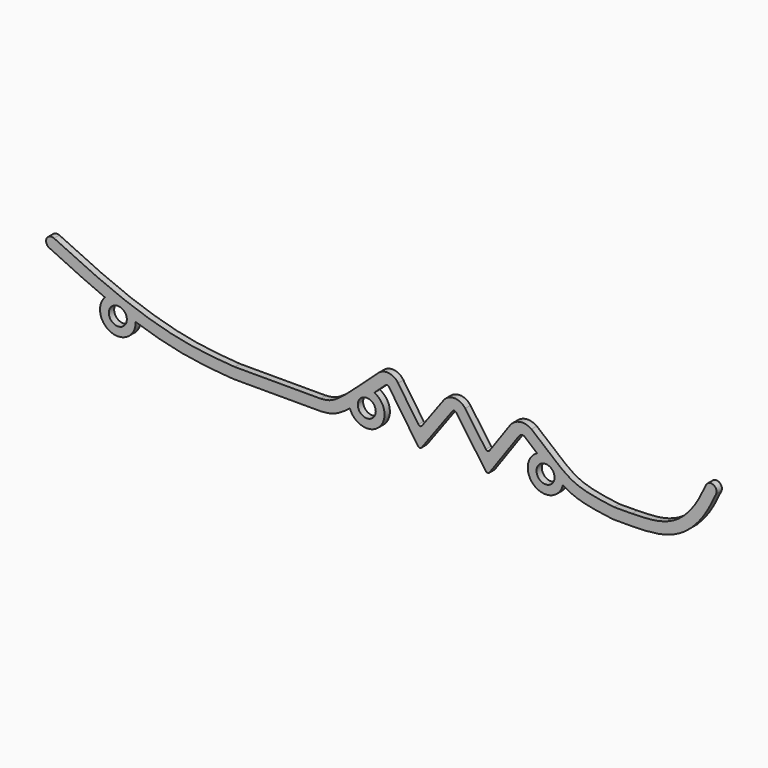
from build123d import *

# Parameters (mm, degrees)
F1_DEPTH = 3


# Not quite as in the source:
# - the dataset's text gives a spline's control points without its knots; the knots are read off the source's solid


with BuildPart() as f1:
    # F0 (on Front) → F1 (new body)
    with BuildSketch(Plane.XZ):
        with BuildLine():
            ThreePointArc((-187.3718851687, -26.828956261), (-187.033666921, -27.7325072413), (-186.9187538398, -28.6904169139))
            ThreePointArc((-186.9187538398, -28.6904169139), (-193.2623391145, -32.02837536), (-192.4209595622, -24.9097293389))
            add(Edge.make_bspline(
                [(-196.7424143686, -23.152832233), (-195.3009482639, -23.7545802912), (-193.8604098699, -24.3410907139), (-192.4209595622, -24.9097293389)],
                knots=[0.2871412748, 0.2871412748, 0.2871412748, 0.2871412748, 0.3367799977, 0.3367799977, 0.3367799977, 0.3367799977], degree=3))
            ThreePointArc((-196.7424143686, -23.152832233), (-193.8049140006, -36.1708043065), (-182.9750665521, -28.3726693011))
            add(Edge.make_bspline(
                [(-187.3718851687, -26.828956261), (-185.9030227612, -27.3646736214), (-184.436648881, -27.8795303136), (-182.9750665521, -28.3726693011)],
                knots=[0.3948765049, 0.3948765049, 0.3948765049, 0.3948765049, 0.4456486133, 0.4456486133, 0.4456486133, 0.4456486133], degree=3))
        make_face()
        with BuildLine():
            ThreePointArc((-192.4209595622, -24.9097293389), (-189.5297427955, -24.9046874975), (-187.3718851687, -26.828956261))
            add(Edge.make_bspline(
                [(-187.3718851687, -26.828956261), (-185.9030227612, -27.3646736214), (-184.436648881, -27.8795303136), (-182.9750665521, -28.3726693011)],
                knots=[0.3948765049, 0.3948765049, 0.3948765049, 0.3948765049, 0.4456486133, 0.4456486133, 0.4456486133, 0.4456486133], degree=3))
            add(Edge.make_bspline(
                [(-182.9750665521, -28.3726693011), (-175.5023077848, -30.893983783), (-159.8116142774, -35.0659243051), (-146.0958365364, -36.1264860321), (-138.8027667999, -36.6904169139)],
                knots=[0.4456486133, 0.4456486133, 0.4456486133, 0.4456486133, 0.7052355763, 1, 1, 1, 1], degree=3))
            Line((-138.8027667999, -36.6904169139), (-99.5722308103, -36.6904169139))
            add(Edge.make_bspline(
                [(-99.5722308103, -36.6904169139), (-97.1488396371, -36.5171262587), (-93.437582007, -36.2517434872), (-88.3445479856, -32.6745172269), (-86.5482922018, -31.2537858599)],
                knots=[0, 0, 0, 0, 0.2792123022, 0.4275945207, 0.4275945207, 0.4275945207, 0.4275945207], degree=3))
            add(Edge.make_bspline(
                [(-86.5482922018, -31.2537858599), (-85.3644963963, -30.3174738669), (-84.1681526298, -29.3032539765), (-82.9986194343, -28.2739371873)],
                knots=[0.4275945207, 0.4275945207, 0.4275945207, 0.4275945207, 0.525383627, 0.525383627, 0.525383627, 0.525383627], degree=3))
            ThreePointArc((-82.9986194343, -28.2739371873), (-81.6948810352, -25.6940829809), (-79.0031430156, -24.6405517881))
            add(Edge.make_bspline(
                [(-79.0031430156, -24.6405517881), (-78.3110296993, -23.9970089125), (-77.0975140376, -22.8616033885), (-76.0302528236, -21.8746017864), (-75.5683654158, -21.449680361)],
                knots=[0.6417671814, 0.6417671814, 0.6417671814, 0.6417671814, 0.7062274661, 0.7602679755, 0.7602679755, 0.7602679755, 0.7602679755], degree=3))
            add(Edge.make_bspline(
                [(-75.5683654158, -21.449680361), (-73.5193617227, -19.5646634603), (-71.9588231198, -18.1752905296), (-70.3982845169, -16.785917599)],
                knots=[0.7602679755, 0.7602679755, 0.7602679755, 0.7602679755, 1, 1, 1, 1], degree=3))
            ThreePointArc((-70.3982845169, -16.785917599), (-69.6491042381, -16.6293438224), (-69.0086394035, -17.0483798986))
            Line((-69.0086394035, -17.0483798986), (-55.9052212397, -36.2540083208))
            ThreePointArc((-55.9052212397, -36.2540083208), (-55.0960197972, -36.6902749044), (-54.272575908, -36.2815259988))
            Line((-54.272575908, -36.2815259988), (-40.3930651403, -17.342386961))
            ThreePointArc((-40.3930651403, -17.342386961), (-39.5781504306, -16.9335306834), (-38.7701542803, -17.3558950534))
            Line((-38.7701542803, -17.3558950534), (-25.3885500453, -36.2680179065))
            ThreePointArc((-25.3885500453, -36.2680179065), (-24.5722308103, -36.6904169139), (-23.7559115754, -36.2680179065))
            Line((-23.7559115754, -36.2680179065), (-10.4562424914, -17.4716933997))
            ThreePointArc((-10.4562424914, -17.4716933997), (-9.4181270946, -16.7173031992), (-8.1352483096, -16.7490864451))
            add(Edge.make_bspline(
                [(-8.1352483096, -16.7490864451), (-6.2116153231, -18.3881130209), (-4.2879823366, -20.0271395967), (-2.3503080936, -21.6557478958)],
                knots=[0, 0, 0, 0, 0.1782199485, 0.1782199485, 0.1782199485, 0.1782199485], degree=3))
            add(Edge.make_bspline(
                [(-2.3503080936, -21.6557478958), (-1.1586889347, -22.6572995543), (0.0382405284, -23.654911094), (1.2437459941, -24.6461594447)],
                knots=[0.1782199485, 0.1782199485, 0.1782199485, 0.1782199485, 0.287820572, 0.287820572, 0.287820572, 0.287820572], degree=3))
            ThreePointArc((1.2437459941, -24.6461594447), (3.9839142587, -25.5235519711), (5.4499310756, -27.9992608506))
            add(Edge.make_bspline(
                [(5.4499310756, -27.9992608506), (6.6628177887, -28.912722829), (7.9128100695, -29.7882065236), (9.2299726213, -30.5923358418)],
                knots=[0.4134276061, 0.4134276061, 0.4134276061, 0.4134276061, 0.5193985301, 0.5193985301, 0.5193985301, 0.5193985301], degree=3))
            add(Edge.make_bspline(
                [(9.2299726213, -30.5923358418), (10.6399819271, -31.4531482148), (16.9397095444, -34.7536327935), (25.2829770933, -35.8516074071), (31.6569060087, -36.6904169139)],
                knots=[0.5193985301, 0.5193985301, 0.5193985301, 0.5193985301, 0.6328393417, 1, 1, 1, 1], degree=3))
            Line((31.6569060087, -36.6904169139), (40.4641851783, -36.6904169139))
            add(Edge.make_bspline(
                [(78.1804878265, -11.6904169139), (76.5395495118, -15.1670466828), (73.1841016711, -22.2761803695), (64.3949954787, -32.0439101559), (52.9263003092, -36.4114346294), (44.6473865624, -36.5967699634), (40.4641851783, -36.6904169139)],
                knots=[0, 0, 0, 0, 0.2448292341, 0.5006353484, 0.7476791079, 1, 1, 1, 1], degree=3))
            ThreePointArc((78.1804878265, -11.6904169139), (76.9867529891, -8.3625050854), (73.6588411606, -9.5562399228))
            add(Edge.make_bspline(
                [(73.6588411606, -9.5562399228), (73.2399424738, -10.4437538725), (72.4166263504, -12.1876945949), (71.1668490557, -14.6995676036), (70.0679787245, -16.7013682285), (69.127277271, -18.2498793256), (68.1382322944, -19.7615171938), (66.777587452, -21.6103262264), (64.9749535667, -23.6915886956), (63.364796253, -25.2471128345), (62.0324117592, -26.3516753747), (61.0208567028, -27.100178839), (59.9879411601, -27.7728309001), (58.5589122141, -28.5888350872), (56.686329422, -29.45622639), (54.7010409101, -30.1341176805), (53.0508363128, -30.5677354982), (51.7873583013, -30.8392065119), (50.4880617372, -31.0606922676), (48.6991336654, -31.2977033298), (46.3658177811, -31.4959214227), (43.4269791424, -31.6226668954), (41.3884619487, -31.6684729316), (40.3522810587, -31.6916693239)],
                knots=[0, 0, 0, 0, 0.0625, 0.125, 0.1875, 0.21875, 0.25, 0.3125, 0.375, 0.4375, 0.46875, 0.5, 0.53125, 0.5625, 0.625, 0.6875, 0.71875, 0.75, 0.78125, 0.8125, 0.875, 0.9375, 1, 1, 1, 1], degree=3))
            Line((40.3522810587, -31.6916693239), (32.3092815115, -31.733158982))
            add(Edge.make_bspline(
                [(-4.8924846752, -12.9432377867), (-3.5432859724, -14.0928190973), (-1.5257519684, -15.811831435), (1.1659958432, -18.0823284028), (2.8524705495, -19.4906139398), (4.2049197686, -20.6086915314), (5.2239262854, -21.4447485184), (6.2375194245, -22.2694933419), (7.5705181247, -23.3340734509), (9.2205919144, -24.5943632283), (11.2048735712, -25.9620365451), (12.8907783422, -26.9628309107), (14.2788914618, -27.6719197), (15.1686099706, -28.0759238998), (15.8956935911, -28.3740988375), (16.6488517668, -28.6617908728), (17.6351494832, -29.0009203407), (18.8866100057, -29.3761933824), (20.6384514215, -29.83619547), (22.9707137683, -30.3404508515), (25.952826553, -30.8548339449), (29.0754850071, -31.307522717), (31.2242781263, -31.5903724579), (32.3092815115, -31.733158982)],
                knots=[0, 0, 0, 0, 0.125, 0.1875, 0.25, 0.28125, 0.3125, 0.34375, 0.375, 0.4375, 0.5, 0.5625, 0.59375, 0.625, 0.640625, 0.65625, 0.6875, 0.71875, 0.75, 0.8125, 0.875, 0.9375, 1, 1, 1, 1], degree=3))
            ThreePointArc((-4.8924846752, -12.9432377867), (-10.0554611604, -11.7626049689), (-14.5378386662, -14.5836884368))
            Line((-14.5378386662, -14.5836884368), (-23.7559115754, -27.6115230869))
            ThreePointArc((-23.7559115754, -27.6115230869), (-24.5722308103, -28.0339220944), (-25.3885500453, -27.6115230869))
            Line((-25.3885500453, -27.6115230869), (-34.6885581054, -14.4678900905))
            ThreePointArc((-34.6885581054, -14.4678900905), (-39.5365350073, -11.9337038708), (-44.4260232659, -14.3868415364))
            Line((-44.4260232659, -14.3868415364), (-54.1266517397, -27.6237311136))
            ThreePointArc((-54.1266517397, -27.6237311136), (-54.9500956289, -28.0324800192), (-55.7592970713, -27.5962134356))
            Line((-55.7592970713, -27.5962134356), (-64.8783708708, -14.2304228642))
            ThreePointArc((-64.8783708708, -14.2304228642), (-69.0304093882, -11.6129272107), (-73.7230803639, -13.0515190429))
            add(Edge.make_bspline(
                [(-99.9288577209, -31.703151406), (-99.3863961349, -31.6643613317), (-98.3965802024, -31.5922292495), (-97.1319214024, -31.4272942541), (-96.1594574741, -31.201702718), (-95.3483085696, -30.9300596969), (-94.8112663863, -30.710060858), (-94.3539289594, -30.4949857761), (-93.9982018206, -30.3133639271), (-93.6156708049, -30.1025456555), (-93.0687035093, -29.7808932287), (-92.3281895703, -29.3085902723), (-91.0519242487, -28.4215203374), (-89.332054283, -27.1036339084), (-87.178514326, -25.3018894715), (-85.0190992997, -23.3880538784), (-82.9255629837, -21.4647591126), (-81.2895574049, -19.9359308439), (-80.070250058, -18.8007049841), (-78.9297096685, -17.7461174963), (-77.6330362977, -16.5587924321), (-76.2352457002, -15.2946646056), (-74.9473734494, -14.1415206842), (-74.1299248932, -13.4137393526), (-73.7230803639, -13.0515190429)],
                knots=[0, 0, 0, 0, 0.0625, 0.125, 0.1875, 0.21875, 0.25, 0.265625, 0.28125, 0.296875, 0.3125, 0.34375, 0.375, 0.4375, 0.5, 0.5625, 0.625, 0.6875, 0.71875, 0.75, 0.8125, 0.875, 0.9375, 1, 1, 1, 1], degree=3))
            Line((-99.9288577209, -31.703151406), (-138.4172963851, -31.705297802))
            add(Edge.make_bspline(
                [(-219.6674946911, -7.1772339179), (-216.0240876916, -8.9145167991), (-208.764438143, -12.375995051), (-199.7744557158, -16.4601389826), (-192.6447117871, -19.4586435844), (-187.336731936, -21.5403994921), (-182.0543420253, -23.4344540573), (-176.8177029617, -25.1356369287), (-171.6569305627, -26.6331260232), (-166.6001394839, -27.9175156957), (-161.6761758195, -28.9808889044), (-156.9164876505, -29.8100414152), (-152.2472369107, -30.4484360928), (-146.0972696954, -31.1109438642), (-141.5100499323, -31.4661530663), (-138.4172963851, -31.705297802)],
                knots=[0, 0, 0, 0, 0.125, 0.25, 0.3125, 0.375, 0.4375, 0.5, 0.5625, 0.625, 0.6875, 0.75, 0.8125, 0.875, 1, 1, 1, 1], degree=3))
            ThreePointArc((-219.6674946911, -7.1772339179), (-223.0000949303, -8.3578166747), (-221.8195121735, -11.6904169139))
            add(Edge.make_bspline(
                [(-221.8195121735, -11.6904169139), (-213.4501319292, -15.6811818839), (-205.0807516849, -19.6719468538), (-196.7424143686, -23.152832233)],
                knots=[0, 0, 0, 0, 0.2871412748, 0.2871412748, 0.2871412748, 0.2871412748], degree=3))
            add(Edge.make_bspline(
                [(-196.7424143686, -23.152832233), (-195.3009482639, -23.7545802912), (-193.8604098699, -24.3410907139), (-192.4209595622, -24.9097293389)],
                knots=[0.2871412748, 0.2871412748, 0.2871412748, 0.2871412748, 0.3367799977, 0.3367799977, 0.3367799977, 0.3367799977], degree=3))
        make_face()
        with BuildLine():
            add(Edge.make_bspline(
                [(-86.5482922018, -31.2537858599), (-85.3644963963, -30.3174738669), (-84.1681526298, -29.3032539765), (-82.9986194343, -28.2739371873)],
                knots=[0.4275945207, 0.4275945207, 0.4275945207, 0.4275945207, 0.525383627, 0.525383627, 0.525383627, 0.525383627], degree=3))
            ThreePointArc((-86.5482922018, -31.2537858599), (-73.641783167, -34.6577563536), (-75.5683654158, -21.449680361))
            add(Edge.make_bspline(
                [(-79.0031430156, -24.6405517881), (-78.3110296993, -23.9970089125), (-77.0975140376, -22.8616033885), (-76.0302528236, -21.8746017864), (-75.5683654158, -21.449680361)],
                knots=[0.6417671814, 0.6417671814, 0.6417671814, 0.6417671814, 0.7062274661, 0.7602679755, 0.7602679755, 0.7602679755, 0.7602679755], degree=3))
            ThreePointArc((-79.0031430156, -24.6405517881), (-76.1180178643, -25.8149723989), (-74.9200905915, -28.6904169139))
            ThreePointArc((-74.9200905915, -28.6904169139), (-79.1786070017, -32.7350455627), (-82.9986194343, -28.2739371873))
        make_face()
        with BuildLine():
            add(Edge.make_bspline(
                [(-2.3503080936, -21.6557478958), (-1.1586889347, -22.6572995543), (0.0382405284, -23.654911094), (1.2437459941, -24.6461594447)],
                knots=[0.1782199485, 0.1782199485, 0.1782199485, 0.1782199485, 0.287820572, 0.287820572, 0.287820572, 0.287820572], degree=3))
            ThreePointArc((-2.3503080936, -21.6557478958), (-3.428192795, -35.0238209142), (9.2299726213, -30.5923358418))
            add(Edge.make_bspline(
                [(5.4499310756, -27.9992608506), (6.6628177887, -28.912722829), (7.9128100695, -29.7882065236), (9.2299726213, -30.5923358418)],
                knots=[0.4134276061, 0.4134276061, 0.4134276061, 0.4134276061, 0.5193985301, 0.5193985301, 0.5193985301, 0.5193985301], degree=3))
            ThreePointArc((5.4499310756, -27.9992608506), (5.4944617341, -28.3435645209), (5.5093417337, -28.6904169139))
            ThreePointArc((5.5093417337, -28.6904169139), (-1.3271737656, -31.6294356911), (1.2437459941, -24.6461594447))
        make_face()
    extrude(amount=F1_DEPTH)


solid = f1.part
